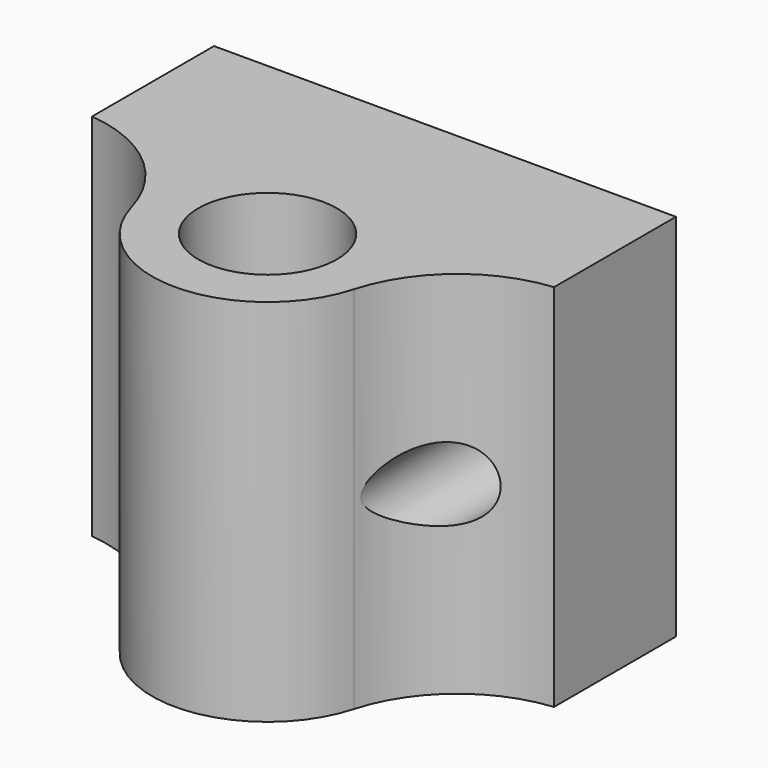
from build123d import *

# Parameters (mm, degrees)
F1_DEPTH    = 40
F2_T1_DEPTH = 40
F3_R        = 4
F4_DEPTH    = 30


# Not quite as in the source:
# - a fillet or chamfer that OpenCascade refuses, or shapes differently, is made with other operations: its cross-section is extruded or revolved along the edge and cut away or added


with BuildPart() as f1:
    # F0 (on Top) → F1 (new body)
    with BuildSketch(Plane.XY):
        with BuildLine():
            Line((10, 7.5), (0, 7.5))
            Line((0, 7.5), (-10, 7.5))
            ThreePointArc((-10, 7.5), (-3.9528470752, -11.8585412256), (12.5, 0))
            ThreePointArc((12.5, 0), (11.8585412256, 3.9528470752), (10, 7.5))
        make_face()
        with BuildLine():
            ThreePointArc((0, 7.5), (5.3033008589, 5.3033008589), (7.5, 0))
            ThreePointArc((7.5, 0), (-5.3033008589, -5.3033008589), (0, 7.5))
        make_face(mode=Mode.SUBTRACT)
        with BuildLine():
            Line((0, 12.5), (0, 7.5))
            Line((0, 7.5), (10, 7.5))
            ThreePointArc((10, 7.5), (5.5901699437, 11.1803398875), (0, 12.5))
        make_face()
        with BuildLine():
            ThreePointArc((0, 12.5), (5.5901699437, 11.1803398875), (10, 7.5))
            Line((10, 7.5), (25, 7.5))
            Line((25, 7.5), (25, 24))
            Line((25, 24), (0, 24))
            Line((0, 24), (0, 12.5))
        make_face()
        with BuildLine():
            ThreePointArc((-10, 7.5), (-5.5901699437, 11.1803398875), (0, 12.5))
            Line((0, 12.5), (0, 24))
            Line((0, 24), (-25, 24))
            Line((-25, 24), (-25, 7.5))
            Line((-25, 7.5), (-10, 7.5))
        make_face()
        with BuildLine():
            Line((-10, 7.5), (0, 7.5))
            Line((0, 7.5), (0, 12.5))
            ThreePointArc((0, 12.5), (-5.5901699437, 11.1803398875), (-10, 7.5))
        make_face()
    extrude(amount=F1_DEPTH)

    # F2: fillet of radius 15 on 2 edges, made by hand

    # F2_s2 → F2_t1 (join)
    with BuildSketch(Plane.XY):
        with BuildLine():
            ThreePointArc((12.0354995182, -3.375907485), (16.8376373335, 4.064804959), (25, 7.5))
            Line((25, 7.5), (10, 7.5))
            ThreePointArc((10, 7.5), (12.2866655631, 2.2995324178), (12.0354995182, -3.375907485))
        make_face()
        with BuildLine():
            ThreePointArc((-25, 7.5), (-16.8376373335, 4.064804959), (-12.0354995182, -3.375907485))
            ThreePointArc((-12.0354995182, -3.375907485), (-12.2866655631, 2.2995324178), (-10, 7.5))
            Line((-10, 7.5), (-25, 7.5))
        make_face()
    extrude(amount=F2_T1_DEPTH)

    # F3 (on Front) → F4 (cut, symmetric)
    with BuildSketch(Plane.XZ):
        with Locations((16.25, 20)):
            Circle(F3_R)
        with Locations((-16.25, 20)):
            Circle(F3_R)
    extrude(amount=F4_DEPTH, both=True, mode=Mode.SUBTRACT)


solid = f1.part
